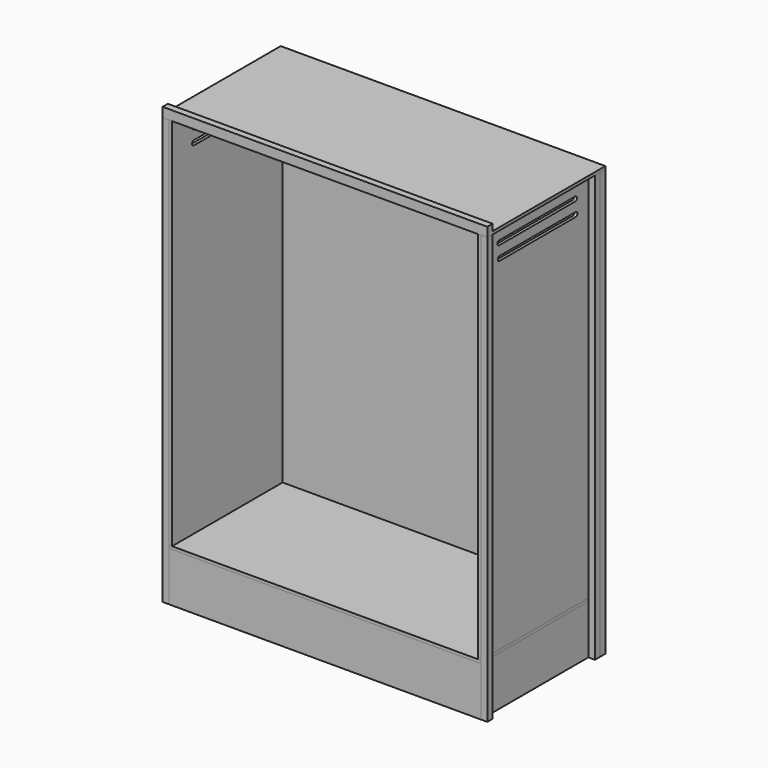
from build123d import *

# Parameters (mm, degrees)
F0_W      = 1900
F0_H      = 860
F0_W_2    = 425
F0_H_2    = 225
F0_H_3    = 250
F1_DEPTH  = 300
F2_W      = 1900
F2_H      = 860
F3_DEPTH  = 18
F4_W      = 40
F4_H      = 2600
F5_DEPTH  = 40
F6_W      = 860
F6_H      = 2282
F7_DEPTH  = 18
F8_W      = 40
F8_H      = 2600
F9_DEPTH  = 40
F10_W     = 860
F10_H     = 2282
F11_DEPTH = 18
F12_W     = 100
F12_H     = 2600
F13_DEPTH = 40
F14_W     = 1874
F14_H     = 2282
F15_DEPTH = 18
F16_W     = 1980
F16_H     = 900
F17_DEPTH = 18
F18_W     = 40
F18_H     = 100
F19_DEPTH = 1780
F20_W     = 40
F20_H     = 40
F21_DEPTH = 1980
F23_DEPTH = 1940.001
F25_DEPTH = 25


with BuildPart() as f1:
    # F0 (on Top) → F1 (new body)
    with BuildSketch(Plane.XY):
        with Locations((950, 430)):
            Rectangle(F0_W, F0_H)
        with Locations((252.5, 152.5)):
            Rectangle(F0_W_2, F0_H_2, mode=Mode.SUBTRACT)
        with Locations((717.5, 152.5)):
            Rectangle(F0_W_2, F0_H_2, mode=Mode.SUBTRACT)
        with Locations((1182.5, 152.5)):
            Rectangle(F0_W_2, F0_H_2, mode=Mode.SUBTRACT)
        with Locations((1647.5, 152.5)):
            Rectangle(F0_W_2, F0_H_2, mode=Mode.SUBTRACT)
        with Locations((252.5, 430)):
            Rectangle(F0_W_2, F0_H_3, mode=Mode.SUBTRACT)
        with Locations((717.5, 430)):
            Rectangle(F0_W_2, F0_H_3, mode=Mode.SUBTRACT)
        with Locations((252.5, 707.5)):
            Rectangle(F0_W_2, F0_H_2, mode=Mode.SUBTRACT)
        with Locations((717.5, 707.5)):
            Rectangle(F0_W_2, F0_H_2, mode=Mode.SUBTRACT)
        with Locations((1182.5, 430)):
            Rectangle(F0_W_2, F0_H_3, mode=Mode.SUBTRACT)
        with Locations((1647.5, 430)):
            Rectangle(F0_W_2, F0_H_3, mode=Mode.SUBTRACT)
        with Locations((1182.5, 707.5)):
            Rectangle(F0_W_2, F0_H_2, mode=Mode.SUBTRACT)
        with Locations((1647.5, 707.5)):
            Rectangle(F0_W_2, F0_H_2, mode=Mode.SUBTRACT)
    extrude(amount=F1_DEPTH)


with BuildPart() as f3:
    # F2 (on face) → F3 (new body)
    with BuildSketch(Plane.XY.offset(300)):
        with Locations((950, 430)):
            Rectangle(F2_W, F2_H)
    extrude(amount=F3_DEPTH)


with BuildPart() as f5:
    # F4 (on face) → F5 (new body)
    with BuildSketch(Plane(origin=(0, 0, 0), x_dir=(0, -1, 0), z_dir=(-1, 0, 0))):
        with Locations((-840, 1300)):
            Rectangle(F4_W, F4_H)
    extrude(amount=F5_DEPTH)


with BuildPart() as f5b:
    # F4 (on face) → F5, piece 2 (new body)
    with BuildSketch(Plane(origin=(0, 0, 0), x_dir=(0, -1, 0), z_dir=(-1, 0, 0))):
        with Locations((-20, 1300)):
            Rectangle(F4_W, F4_H)
    extrude(amount=F5_DEPTH)


with BuildPart() as f7:
    # F6 (on face) → F7 (new body)
    with BuildSketch(Plane.YZ):
        with Locations((430, 1459)):
            Rectangle(F6_W, F6_H)
    extrude(amount=F7_DEPTH)

    # F24 (on face) → F25 (cut)
    with BuildSketch(Plane(origin=(0, 0, 0), x_dir=(0, -1, 0), z_dir=(-1, 0, 0))):
        with BuildLine():
            Line((-166.1425959082, 2516), (-693.8574040918, 2516))
            ThreePointArc((-693.8574040918, 2516), (-707.8574040918, 2502), (-693.8574040918, 2488))
            Line((-693.8574040918, 2488), (-166.1425959082, 2488))
            ThreePointArc((-166.1425959082, 2488), (-152.1425959082, 2502), (-166.1425959082, 2516))
        make_face()
        with BuildLine():
            Line((-166.1425959082, 2430), (-693.8574040918, 2430))
            ThreePointArc((-693.8574040918, 2430), (-707.8574040918, 2416), (-693.8574040918, 2402))
            Line((-693.8574040918, 2402), (-166.1425959082, 2402))
            ThreePointArc((-166.1425959082, 2402), (-152.1425959082, 2416), (-166.1425959082, 2430))
        make_face()
    extrude(amount=-F25_DEPTH, mode=Mode.SUBTRACT)


with BuildPart() as f9:
    # F8 (on face) → F9 (new body)
    with BuildSketch(Plane.YZ.offset(1900)):
        with Locations((20, 1300)):
            Rectangle(F8_W, F8_H)
    extrude(amount=F9_DEPTH)


with BuildPart() as f9b:
    # F8 (on face) → F9, piece 2 (new body)
    with BuildSketch(Plane.YZ.offset(1900)):
        with Locations((840, 1300)):
            Rectangle(F8_W, F8_H)
    extrude(amount=F9_DEPTH)


with BuildPart() as f11:
    # F10 (on face) → F11 (new body)
    with BuildSketch(Plane(origin=(1900, 0, 0), x_dir=(0, -1, 0), z_dir=(-1, 0, 0))):
        with Locations((-430, 1459)):
            Rectangle(F10_W, F10_H)
    extrude(amount=F11_DEPTH)

    # F22 (on face) → F23 (cut, through all)
    with BuildSketch(Plane.YZ.offset(1900)):
        with BuildLine():
            ThreePointArc((140, 2515.121550531), (126.5222263626, 2501.6437768936), (140, 2488.1660032562))
            Line((140, 2488.1660032562), (720, 2488.1660032562))
            ThreePointArc((720, 2488.1660032562), (733.4777736374, 2501.6437768936), (720, 2515.121550531))
            Line((720, 2515.121550531), (140, 2515.121550531))
        make_face()
        with BuildLine():
            ThreePointArc((142.9552948475, 2430.2057933518), (129.4775212101, 2416.7280197144), (142.9552948475, 2403.2502460769))
            Line((142.9552948475, 2403.2502460769), (722.9552948475, 2403.2502460769))
            ThreePointArc((722.9552948475, 2403.2502460769), (736.4330684849, 2416.7280197144), (722.9552948475, 2430.2057933518))
            Line((722.9552948475, 2430.2057933518), (142.9552948475, 2430.2057933518))
        make_face()
    extrude(amount=-F23_DEPTH, mode=Mode.SUBTRACT)


with BuildPart() as f13:
    # F12 (on face) → F13 (new body)
    with BuildSketch(Plane(origin=(0, 860, 0), x_dir=(-1, 0, 0), z_dir=(0, 1, 0))):
        with Locations((-1890, 1300)):
            Rectangle(F12_W, F12_H)
    extrude(amount=F13_DEPTH)


with BuildPart() as f13b:
    # F12 (on face) → F13, piece 2 (new body)
    with BuildSketch(Plane(origin=(0, 860, 0), x_dir=(-1, 0, 0), z_dir=(0, 1, 0))):
        with Locations((-10, 1300)):
            Rectangle(F12_W, F12_H)
    extrude(amount=F13_DEPTH)


with BuildPart() as f15:
    # F14 (on face) → F15 (new body)
    with BuildSketch(Plane.XZ.offset(-860)):
        with Locations((955, 1459)):
            Rectangle(F14_W, F14_H)
    extrude(amount=F15_DEPTH)


with BuildPart() as f17:
    # F16 (on face) → F17 (new body)
    with BuildSketch(Plane.XY.offset(2600)):
        with Locations((950, 450)):
            Rectangle(F16_W, F16_H)
    extrude(amount=F17_DEPTH)

    # F20 (on face) → F21 (join)
    with BuildSketch(Plane.YZ.offset(1940)):
        with Locations((20, 2638)):
            Rectangle(F20_W, F20_H)
    extrude(amount=-F21_DEPTH)


with BuildPart() as f19:
    # F18 (on face) → F19 (new body, through all)
    with BuildSketch(Plane.YZ.offset(60)):
        with Locations((880, 1460)):
            Rectangle(F18_W, F18_H)
    extrude(amount=F19_DEPTH)


solid = Compound([f1.part, f3.part, f5.part, f5b.part, f7.part, f9.part, f9b.part, f11.part, f13.part, f13b.part, f15.part, f17.part, f19.part])
